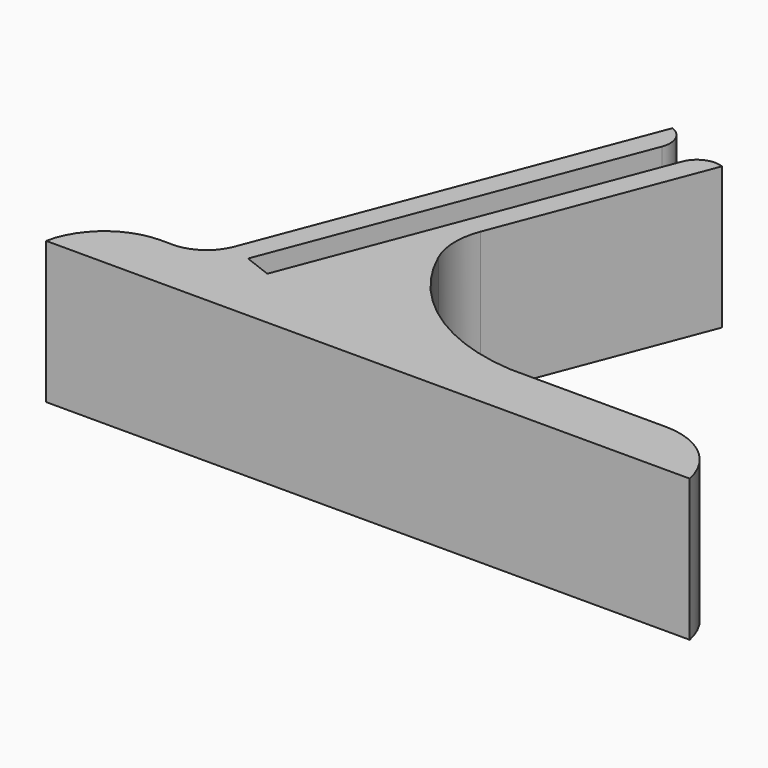
from build123d import *

# Parameters (mm, degrees)
F1_DEPTH    = 10
F2_T1_DEPTH = 10
F2_T3_DEPTH = 34.4948974279
F2_T5_DEPTH = 34.4948974279
F3_R        = 3
F4_R        = 1.59999


# Not quite as in the source:
# - a fillet or chamfer that OpenCascade refuses, or shapes differently, is made with other operations: its cross-section is extruded or revolved along the edge and cut away or added
# - a fillet or chamfer is up to 0.001 mm smaller than in the source, because OpenCascade refuses the exact size


with BuildPart() as f1:
    # F0 (on Top) → F1 (new body)
    with BuildSketch(Plane.XY):
        with BuildLine():
            Line((-7.7799167484, 4), (-7.7799167484, 0))
            Line((-7.7799167484, 0), (37.5679595768, 0))
            Line((37.5679595768, 0), (37.5679595768, 4))
            Line((37.5679595768, 4), (21.6996651143, 4))
            ThreePointArc((21.6996651143, 4), (13.9894641382, 7.0819259987), (9.5494964602, 14.0984888306))
            Line((9.5494964602, 14.0984888306), (15.7092516907, 30.1592148483))
            Line((15.7092516907, 30.1592148483), (14.215355652, 30.732167399))
            Line((14.215355652, 30.732167399), (4.170825278, 4.5424172749))
            Line((4.170825278, 4.5424172749), (2.2100867272, 5.2944174977))
            Line((2.2100867272, 5.2944174977), (12.2367563651, 31.4375981759))
            Line((12.2367563651, 31.4375981759), (10.7428603263, 32.0105507266))
            Line((10.7428603263, 32.0105507266), (0, 4))
            Line((0, 4), (-7.7799167484, 4))
        make_face()
    extrude(amount=F1_DEPTH)

    # F2: fillet of radius 5 on 3 edges, made by hand

    # F2_s2 → F2_t1 (join)
    with BuildSketch(Plane.XY):
        with BuildLine():
            ThreePointArc((10.2974988853, 11.9526797446), (9.8650823787, 13.8567183835), (10.1948614585, 15.7811905013))
            Line((10.1948614585, 15.7811905013), (9.5494964602, 14.0984888306))
            ThreePointArc((9.5494964602, 14.0984888306), (9.8781857469, 13.0097891124), (10.2974988853, 11.9526797446))
        make_face()
    extrude(amount=F2_T1_DEPTH)

    # F2_s4 → F2_t3 (cut)
    with BuildSketch(Plane.XY.offset(-12.2474487139)):
        with BuildLine():
            ThreePointArc((-2.8809372628, 4), (-6.043214923, 2.8729833462), (-7.7799167484, 0))
            Line((-7.7799167484, 0), (-7.7799167484, 4))
            Line((-7.7799167484, 4), (-2.8809372628, 4))
        make_face()
    extrude(amount=F2_T3_DEPTH, mode=Mode.SUBTRACT)

    # F2_s6 → F2_t5 (cut)
    with BuildSketch(Plane.XY.offset(-12.2474487139)):
        with BuildLine():
            ThreePointArc((32.6689800913, 4), (35.8312577514, 2.8729833462), (37.5679595768, 0))
            Line((37.5679595768, 0), (37.5679595768, 4))
            Line((37.5679595768, 4), (32.6689800913, 4))
        make_face()
    extrude(amount=F2_T5_DEPTH, mode=Mode.SUBTRACT)

    # F3
    f3_edges = [f1.edges().sort_by_distance(p)[0] for p in [
        (0, 4, 5),
    ]]
    fillet(f3_edges, radius=F3_R)

    # F4 (radius 1.6 in the source; OpenCascade refuses exactly that, so slightly less here)
    f4_edges = [f1.edges().sort_by_distance(p)[0] for p in [
        (12.236756, 31.437598, 5),
        (14.215356, 30.732167, 5),
    ]]
    fillet(f4_edges, radius=F4_R)


solid = f1.part
